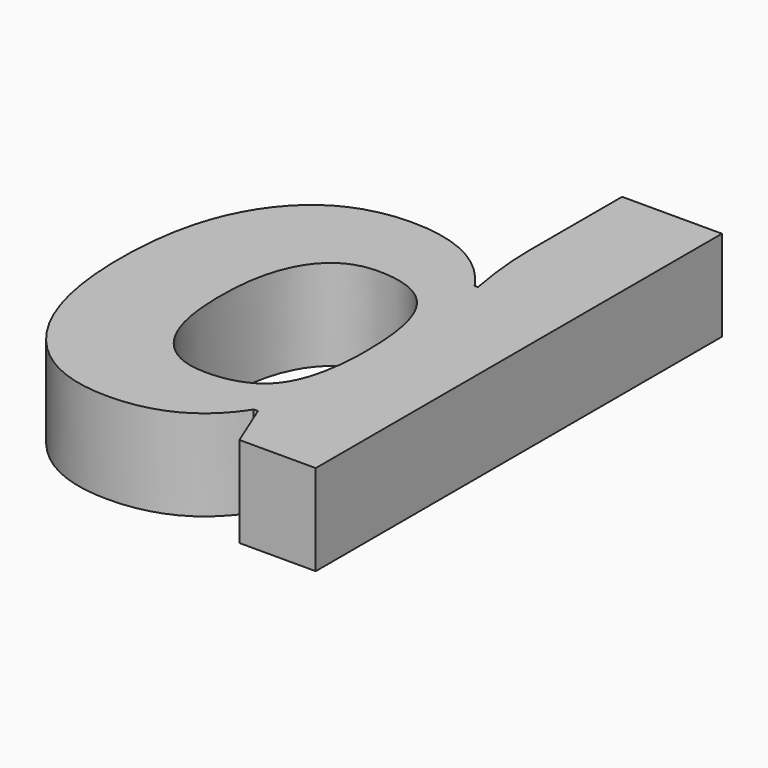
from build123d import *

# Parameters (mm, degrees)
F0_TEXT_SIZE = 73.6177898943
F1_DEPTH     = 10


# Not quite as in the source:
# - Text() gives the source's letters only with a copy of the font that has no kerning and outlines rounded to 1/6400 em; it was checked with that copy


with BuildPart() as f1:
    # F0 (on Top) → F1 (new body)
    with BuildSketch(Plane.XY):
        with Locations((0, 0)):
            Text('d', F0_TEXT_SIZE, font='Open Sans', font_style=FontStyle.BOLD, text_align=(TextAlign.LEFT, TextAlign.BOTTOM))
    extrude(amount=F1_DEPTH)


solid = f1.part
